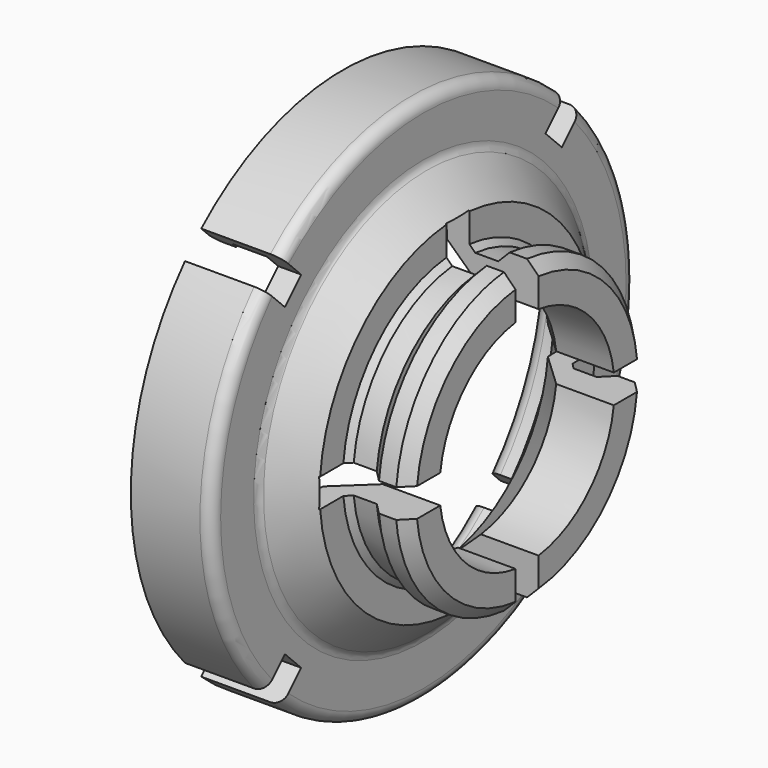
from build123d import *

# Parameters (mm, degrees)
F1_W     = 2.5
F1_H     = 30
F4_DEPTH = 20
F2_W     = 30
F2_H     = 2.5
F5_DEPTH = 20
F6_R     = 1
F8_DEPTH = 13.7
F9_SIZE  = 1


with BuildPart() as f3:
    # F0 (on Front) → F3 (revolve)
    with BuildSketch(Plane.XZ):
        Polygon((-7, 22.9999999304), (-6.9995828196, 21.75), (-5.9995828196, 21.75), (-4.9995828196, 21.75), (-4.9989218824, 21.75), (-1.9995828196, 21.75), (-2, 16.75), (1, 13.75), (1.0601244867, 12.25), (4, 9.5), (9, 9.5), (9.000636667, 13), (5.500636667, 13), (5.500636667, 11.9990898296), (3.500636667, 11.9990898296), (3, 12.4969976023), (3, 15), (0, 18), (0, 23), align=None)
        with BuildLine():
            Line((-5.9995828196, 21.75), (-6.9995828196, 21.75))
            ThreePointArc((-6.9995828196, 21.75), (-6.5667806083, 21.3178286291), (-5.9736431893, 21.1685709655))
            Line((-5.9736431893, 21.1685709655), (-5.9995828196, 21.1685709655))
            Line((-5.9995828196, 21.1685709655), (-5.9995828196, 21.75))
        make_face()
        with BuildLine():
            Line((-4.9995828196, 21.75), (-5.9995828196, 21.75))
            Line((-5.9995828196, 21.75), (-5.9995828196, 21.1685709655))
            Line((-5.9995828196, 21.1685709655), (-5.9736431893, 21.1685709655))
            ThreePointArc((-5.9736431893, 21.1685709655), (-5.4099617873, 21.3308727126), (-4.9995828196, 21.75))
        make_face()
        with BuildLine():
            ThreePointArc((-4.9995828196, 21.75), (-5.4099617873, 21.3308727126), (-5.9736431893, 21.1685709655))
            Line((-5.9736431893, 21.1685709655), (-4.9989218824, 21.1685709655))
            Line((-4.9989218824, 21.1685709655), (-4.9989218824, 21.75))
            Line((-4.9989218824, 21.75), (-4.9995828196, 21.75))
        make_face()
    revolve(axis=Axis((-16.9169774101, 0, 0), (-1, 0, 0)))

    # F1 (on Right) → F4 (cut)
    with BuildSketch(Plane.YZ):
        Rectangle(F1_W, F1_H)
    extrude(amount=F4_DEPTH, mode=Mode.SUBTRACT)

    # F2 (on Right) → F5 (cut)
    with BuildSketch(Plane.YZ):
        Rectangle(F2_W, F2_H)
    extrude(amount=F5_DEPTH, mode=Mode.SUBTRACT)

    # F6
    f6_edges = [f3.edges().sort_by_distance(p)[0] for p in [
        (0, 0, -23),
        (0, 0, -18),
    ]]
    fillet(f6_edges, radius=F6_R)

    # F7 (on Right) → F8 (cut)
    with BuildSketch(Plane.YZ):
        Polygon((-13.2582521472, 15.0260191002), (-16.7937860532, 18.5615530061), (-18.5615530061, 16.7937860532), (-15.0260191002, 13.2582521472), align=None)
        Polygon((18.5615530061, 16.7937860532), (16.7937860532, 18.5615530061), (13.2582521472, 15.0260191002), (15.0260191002, 13.2582521472), align=None)
        Polygon((16.7937860532, -18.5615530061), (18.5615530061, -16.7937860532), (15.0260191002, -13.2582521472), (13.2582521472, -15.0260191002), align=None)
        Polygon((-18.5615530061, -16.7937860532), (-16.7937860532, -18.5615530061), (-13.2582521472, -15.0260191002), (-15.0260191002, -13.2582521472), align=None)
    extrude(amount=-F8_DEPTH, mode=Mode.SUBTRACT)

    # F9
    f9_edges = [f3.edges().sort_by_distance(p)[0] for p in [
        (5.500637, -9.192388, 9.192388),
        (9.000637, -9.192388, 9.192388),
        (9.000637, 9.192388, 9.192388),
        (9.000637, 9.192388, -9.192388),
        (9.000637, -9.192388, -9.192388),
        (5.500637, -9.192388, -9.192388),
        (5.500637, 9.192388, 9.192388),
        (5.500637, 9.192388, -9.192388),
    ]]
    chamfer(f9_edges, length=F9_SIZE)


solid = f3.part
